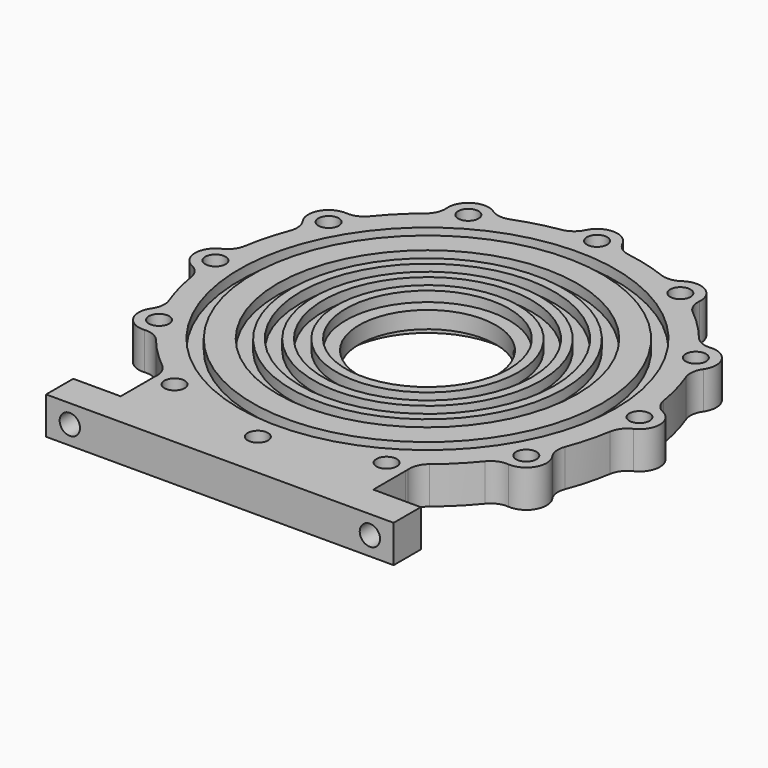
from build123d import *

# Parameters (mm, degrees)
F2_R           = 6
F3_DEPTH       = 11
F4_R           = 3
F5_DEPTH       = 11.001
F6_R           = 6
F8_DEPTH       = 11
F9_R           = 3
F10_DEPTH      = 10.0010001
F14_R          = 1.25
F15_DEPTH      = 1.3299809673
F15_DEPTH_BACK = 43.0588283222
F16_R          = 3
F16_R_2        = 1.25
F17_DEPTH      = 4
F17_DEPTH_BACK = 1.3299809673


with BuildPart() as f1:
    # F0 (on Front) → F1 (revolve)
    with BuildSketch(Plane.XZ):
        Polygon((20.15, 3), (24.05, 3), (24.05, 0), (26.75, 0), (26.75, 3), (30.75, 3), (30.75, 0), (33.45, 0), (33.45, 3), (37.45, 3), (37.45, 0), (40.15, 0), (40.15, 3), (44.15, 3), (44.15, 0), (51.5, 0), (51.5, 3), (55.5, 3), (55.5, 0), (62.5, 0), (62.5, 5.5), (62.5, 11), (55.5, 11), (55.5, 8), (51.5, 8), (51.5, 11), (44.15, 11), (44.15, 8), (40.15, 8), (40.15, 11), (37.45, 11), (37.45, 8), (33.45, 8), (33.45, 11), (30.75, 11), (30.75, 8), (26.75, 8), (26.75, 11), (24.05, 11), (24.05, 8), (20.15, 8), (20.15, 5.5), align=None)
    revolve(axis=Axis((0, 0, 10.994283542), (0, 0, 1)))

    # F2 (on face) → F3 (join, through all)
    with BuildSketch(Plane.XY.offset(11)):
        with Locations((0, 62.5)):
            Circle(F2_R)
        with Locations((-31.25, 54.1265877365)):
            Circle(F2_R)
        with Locations((-54.1265877365, 31.25)):
            Circle(F2_R)
        with Locations((-62.5, 0)):
            Circle(F2_R)
        with Locations((-54.1265877365, -31.25)):
            Circle(F2_R)
        with Locations((-31.25, -54.1265877365)):
            Circle(F2_R)
        with Locations((0, -62.5)):
            Circle(F2_R)
        with Locations((31.25, -54.1265877365)):
            Circle(F2_R)
        with Locations((54.1265877365, -31.25)):
            Circle(F2_R)
        with Locations((62.5, 0)):
            Circle(F2_R)
        with Locations((54.1265877365, 31.25)):
            Circle(F2_R)
        with Locations((31.25, 54.1265877365)):
            Circle(F2_R)
    extrude(amount=-F3_DEPTH)

    # F4 (on face) → F5 (cut, through all)
    with BuildSketch(Plane.XY.offset(11)):
        with Locations((0, 62.5)):
            Circle(F4_R)
        with Locations((-31.25, 54.1265877365)):
            Circle(F4_R)
        with Locations((-54.1265877365, 31.25)):
            Circle(F4_R)
        with Locations((-62.5, 0)):
            Circle(F4_R)
        with Locations((-54.1265877365, -31.25)):
            Circle(F4_R)
        with Locations((-31.25, -54.1265877365)):
            Circle(F4_R)
        with Locations((0, -62.5)):
            Circle(F4_R)
        with Locations((31.25, -54.1265877365)):
            Circle(F4_R)
        with Locations((54.1265877365, -31.25)):
            Circle(F4_R)
        with Locations((62.5, 0)):
            Circle(F4_R)
        with Locations((54.1265877365, 31.25)):
            Circle(F4_R)
        with Locations((31.25, 54.1265877365)):
            Circle(F4_R)
    extrude(amount=-F5_DEPTH, mode=Mode.SUBTRACT)

    # F6
    f6_edges = [f1.edges().sort_by_distance(p)[0] for p in [
        (50.88063, -36.296163, 5.5),
        (56.873714, -25.915837, 5.5),
        (25.915837, -56.873714, 5.5),
        (36.296163, -50.88063, 5.5),
        (62.212, -5.993084, 5.5),
        (62.212, 5.993084, 5.5),
        (-5.993084, -62.212, 5.5),
        (5.993084, -62.212, 5.5),
        (-36.296163, -50.88063, 5.5),
        (-25.915837, -56.873714, 5.5),
        (-56.873714, -25.915837, 5.5),
        (-50.88063, -36.296163, 5.5),
        (-50.88063, 36.296163, 5.5),
        (-56.873714, 25.915837, 5.5),
        (-62.212, 5.993084, 5.5),
        (-62.212, -5.993084, 5.5),
        (-25.915837, 56.873714, 5.5),
        (-36.296163, 50.88063, 5.5),
        (5.993084, 62.212, 5.5),
        (-5.993084, 62.212, 5.5),
        (36.296163, 50.88063, 5.5),
        (25.915837, 56.873714, 5.5),
        (50.88063, 36.296163, 5.5),
        (56.873714, 25.915837, 5.5),
    ]]
    fillet(f6_edges, radius=F6_R)

    # F7 (on face) → F8 (join, through all)
    with BuildSketch(Plane.XY.offset(11)):
        with BuildLine():
            ThreePointArc((-27.8378279418, -59.0618771754), (-33.818, -59.5492601404), (-37.2301720582, -54.6139707016))
            Line((-37.2301720582, -54.6139707016), (-37.2301720582, -66.5))
            Line((-37.2301720582, -66.5), (-51.2301720582, -66.5))
            Line((-51.2301720582, -66.5), (-51.2301720582, -76.5))
            Line((-51.2301720582, -76.5), (0, -76.5))
            Line((0, -76.5), (0, -68.5))
            ThreePointArc((0, -68.5), (-3.2087380697, -67.5699112418), (-5.4226724039, -65.068))
            add(Edge.make_bspline(
                [(-5.4226724039, -65.068), (-5.5429562822, -64.8140046466), (-5.6794959474, -64.5641276478), (-5.8322250803, -64.3202834296), (-6.0006556212, -64.0844289441), (-6.3682583942, -63.6308188923), (-6.5676276573, -63.4131866933), (-6.7810250625, -63.2072998782), (-7.0070826946, -63.0147914154), (-7.4811559513, -62.6590473009), (-7.7291768837, -62.4958076661), (-7.9865042891, -62.3484630373), (-8.2511879389, -62.217870378), (-8.7894669413, -61.9917076194), (-9.0629989157, -61.8959138597), (-9.3398134788, -61.8174289027), (-9.6178952594, -61.7561743685), (-9.8953875984, -61.7116788321)],
                knots=[0, 0, 0, 0, 0, 0, 0.2491872976, 0.2491872976, 0.2491872976, 0.2491872976, 0.5, 0.5, 0.5, 0.5, 0.7508127024, 0.7508127024, 0.7508127024, 0.7508127024, 1, 1, 1, 1, 1, 1], degree=5))
            ThreePointArc((-9.8953875984, -61.7116788321), (-16.1761903189, -60.3703641431), (-22.2861823756, -58.391575378))
            add(Edge.make_bspline(
                [(-22.2861823756, -58.391575378), (-22.5487455587, -58.2913634733), (-22.8201987121, -58.2053705658), (-23.0991696344, -58.1349332508), (-23.3839521528, -58.081127093), (-23.9631968225, -58.0078502862), (-24.2577159169, -57.9886050218), (-24.5542403014, -57.9875455107), (-24.850652547, -58.0049047151), (-25.4390840877, -58.0759515272), (-25.7311099712, -58.1296399304), (-26.0188609528, -58.2012444399), (-26.300335899, -58.2900348214), (-26.8454942647, -58.4990712632), (-27.1092866347, -58.6191119688), (-27.3634760528, -58.7539226899), (-27.6066613708, -58.902052686), (-27.8378279418, -59.0618771754)],
                knots=[0, 0, 0, 0, 0, 0, 0.2491872976, 0.2491872976, 0.2491872976, 0.2491872976, 0.5, 0.5, 0.5, 0.5, 0.7508127024, 0.7508127024, 0.7508127024, 0.7508127024, 1, 1, 1, 1, 1, 1], degree=5))
        make_face()
        with BuildLine():
            Line((0, -68.5), (0, -76.5))
            Line((0, -76.5), (51.2301720582, -76.5))
            Line((51.2301720582, -76.5), (51.2301720582, -66.5))
            Line((51.2301720582, -66.5), (37.2301720582, -66.5))
            Line((37.2301720582, -66.5), (37.2301720582, -54.6139707016))
            ThreePointArc((37.2301720582, -54.6139707016), (33.818, -59.5492601404), (27.8378279418, -59.0618771754))
            add(Edge.make_bspline(
                [(27.8378279418, -59.0618771754), (27.6066613708, -58.902052686), (27.3634760528, -58.7539226899), (27.1092866347, -58.6191119688), (26.8454942647, -58.4990712632), (26.300335899, -58.2900348214), (26.0188609528, -58.2012444399), (25.7311099712, -58.1296399304), (25.4390840877, -58.0759515272), (24.850652547, -58.0049047151), (24.5542403014, -57.9875455107), (24.2577159169, -57.9886050218), (23.9631968225, -58.0078502862), (23.3839521528, -58.081127093), (23.0991696344, -58.1349332508), (22.8201987121, -58.2053705658), (22.5487455587, -58.2913634733), (22.2861823756, -58.391575378)],
                knots=[0, 0, 0, 0, 0, 0, 0.2491872976, 0.2491872976, 0.2491872976, 0.2491872976, 0.5, 0.5, 0.5, 0.5, 0.7508127024, 0.7508127024, 0.7508127024, 0.7508127024, 1, 1, 1, 1, 1, 1], degree=5))
            ThreePointArc((22.2861823756, -58.391575378), (16.1761903189, -60.3703641431), (9.8953875984, -61.7116788321))
            add(Edge.make_bspline(
                [(9.8953875984, -61.7116788321), (9.6178952594, -61.7561743685), (9.3398134788, -61.8174289027), (9.0629989157, -61.8959138597), (8.7894669413, -61.9917076194), (8.2511879389, -62.217870378), (7.9865042891, -62.3484630373), (7.7291768837, -62.4958076661), (7.4811559513, -62.6590473009), (7.0070826946, -63.0147914154), (6.7810250625, -63.2072998782), (6.5676276573, -63.4131866933), (6.3682583942, -63.6308188923), (6.0006556212, -64.0844289441), (5.8322250803, -64.3202834296), (5.6794959474, -64.5641276478), (5.5429562822, -64.8140046466), (5.4226724039, -65.068)],
                knots=[0, 0, 0, 0, 0, 0, 0.2491872976, 0.2491872976, 0.2491872976, 0.2491872976, 0.5, 0.5, 0.5, 0.5, 0.7508127024, 0.7508127024, 0.7508127024, 0.7508127024, 1, 1, 1, 1, 1, 1], degree=5))
            ThreePointArc((5.4226724039, -65.068), (3.2087380697, -67.5699112418), (0, -68.5))
        make_face()
    extrude(amount=-F8_DEPTH)

    # F9 (on face) → F10 (cut, through all)
    with BuildSketch(Plane(origin=(0, -66.5, 0), x_dir=(-1, 0, 0), z_dir=(0, 1, 0))):
        with Locations((-44.2301720582, 5.5)):
            Circle(F9_R)
        with Locations((44.2301720582, 5.5)):
            Circle(F9_R)
    extrude(amount=-F10_DEPTH, mode=Mode.SUBTRACT)

    # F14 (on face) → F15 (cut, two sides)
    with BuildSketch(Plane(origin=(43.9608421181, 43.9608421181, 0), x_dir=(0.7071067812, -0.7071067812, 0), z_dir=(-0.7071067812, -0.7071067812, 0))) as f15_sk:
        with Locations((0, 5.5)):
            Circle(F14_R)
    extrude(amount=-F15_DEPTH, mode=Mode.SUBTRACT)
    extrude(f15_sk.sketch, amount=F15_DEPTH_BACK, mode=Mode.SUBTRACT)

    # F16 (on face) → F17 (cut, two sides)
    with BuildSketch(Plane(origin=(43.9608421181, 43.9608421181, 0), x_dir=(0.7071067812, -0.7071067812, 0), z_dir=(-0.7071067812, -0.7071067812, 0))) as f17_sk:
        with Locations((0, 5.5)):
            Circle(F16_R)
        with Locations((0, 5.5)):
            Circle(F16_R_2, mode=Mode.SUBTRACT)
    extrude(amount=F17_DEPTH, mode=Mode.SUBTRACT)
    extrude(f17_sk.sketch, amount=-F17_DEPTH_BACK, mode=Mode.SUBTRACT)


solid = f1.part
